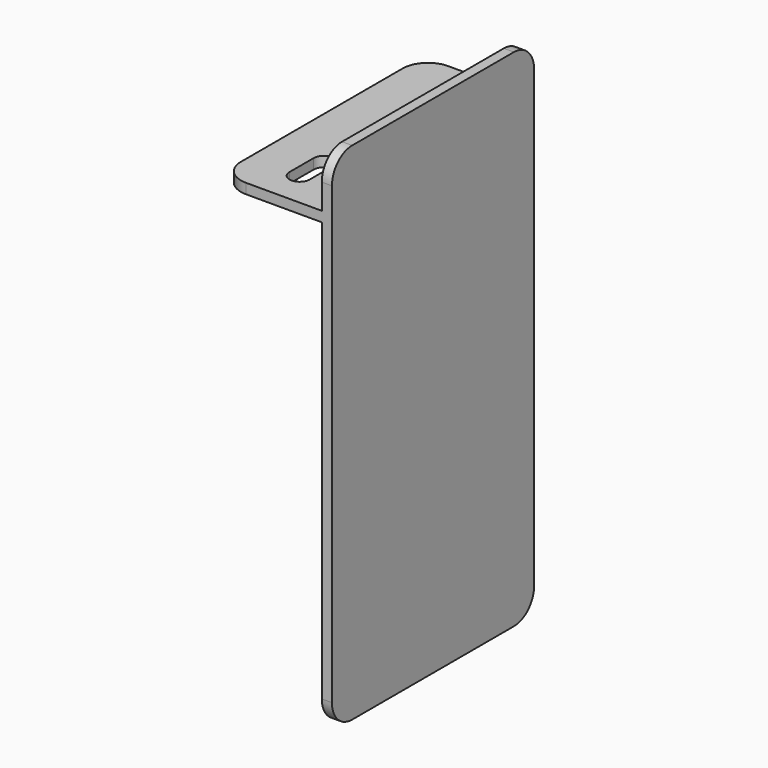
from build123d import *

# Parameters (mm, degrees)
F1_DEPTH = 50
F3_DEPTH = 25
F4_R     = 5


# Not quite as in the source:
# - a feature names something its author has since deleted; it is built from what else it names


with BuildPart() as f1:
    # F0 (on Front) → F1 (new body)
    with BuildSketch(Plane.XZ):
        Polygon((0, 0), (0, -2), (20, -2), (20, -90), (22, -90), (22, 10), (20, 10), (20, 0), align=None)
    extrude(amount=F1_DEPTH)

    # F2 (on face) → F3 (cut)
    with BuildSketch(Plane.XY):
        with BuildLine():
            ThreePointArc((12, -7), (10, -5), (8, -7))
            Line((8, -7), (8, -13))
            ThreePointArc((8, -13), (10, -15), (12, -13))
            Line((12, -13), (12, -7))
        make_face()
        with BuildLine():
            ThreePointArc((8, -43), (10, -45), (12, -43))
            Line((12, -43), (12, -37))
            ThreePointArc((12, -37), (10, -35), (8, -37))
            Line((8, -37), (8, -43))
        make_face()
    extrude(amount=-F3_DEPTH, mode=Mode.SUBTRACT)

    # F4
    f4_edges = [f1.edges().sort_by_distance(p)[0] for p in [
        (21, -50, 10),
        (21, 0, 10),
        (21, -50, -90),
        (21, 0, -90),
        (0, -50, -1),
        (0, 0, -1),
    ]]
    fillet(f4_edges, radius=F4_R)


solid = f1.part
